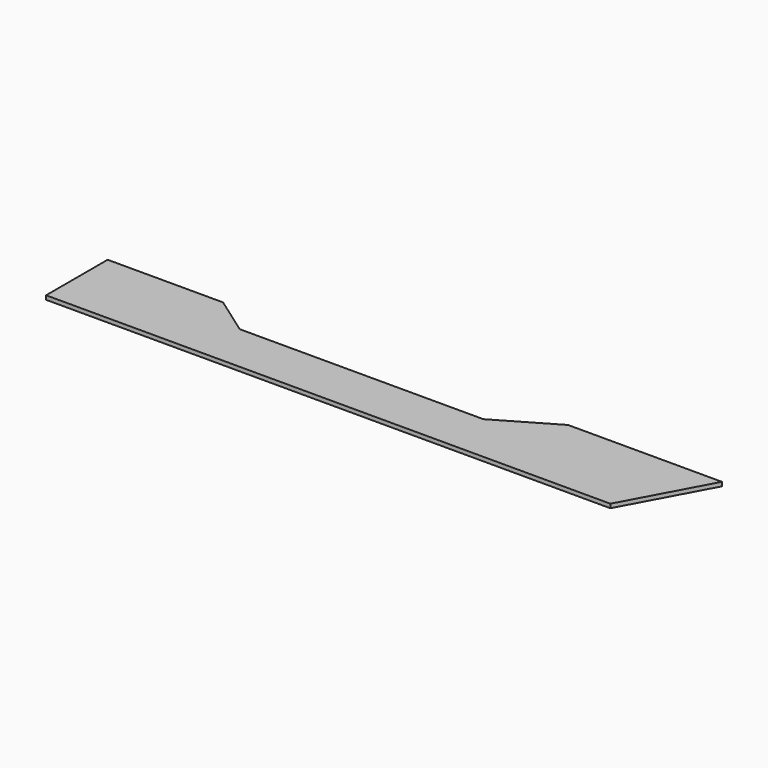
from build123d import *

# Parameters (mm, degrees)
F1_DEPTH = 15.875


# Not quite as in the source:
# - a length typed as a fraction of an inch, garbled in the dataset ("3 / 203.2 mm" for 3/8 in), is restored


with BuildPart() as f1:
    # F0 (on Top) → F1 (new body)
    with BuildSketch(Plane.XY):
        Polygon((0, 304.8), (0, 0), (2235.2, 0), (2413, 330.2), (1803.4, 330.2), (1574.8, 196.85), (609.6, 196.85), (457.2, 304.8), align=None)
    extrude(amount=F1_DEPTH)


solid = f1.part
